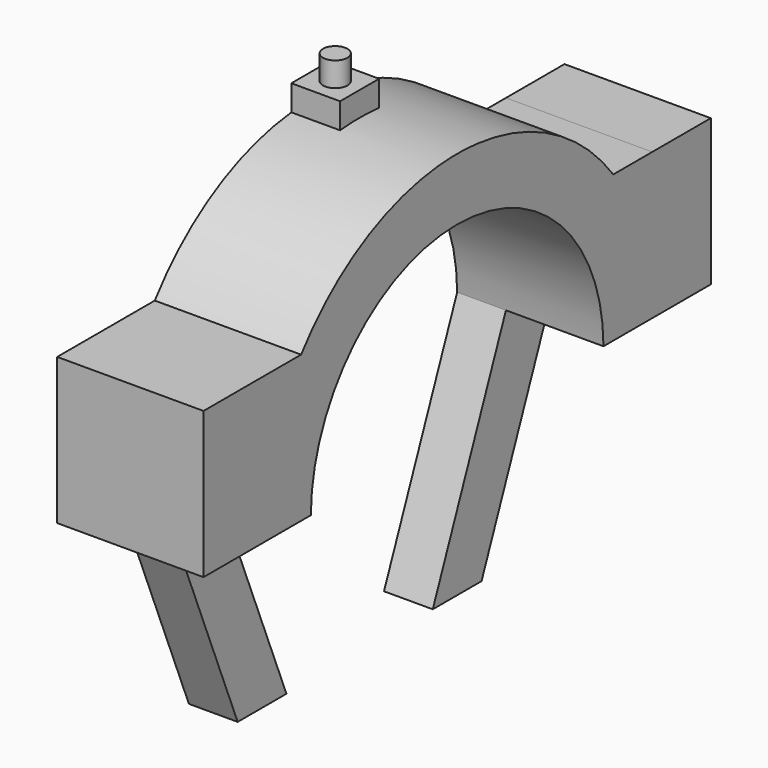
from build123d import *

# Parameters (mm, degrees)
F0_W     = 7.62
F0_H     = 15.24
F1_DEPTH = 5.08
F2_R     = 1.27
F3_DEPTH = 2.54
F4_DEPTH = 15.24


# Not quite as in the source:
# - ends of sketch curves that miss each other by under 0.0002 mm in the source are joined


with BuildPart() as f1:
    # F0 (on Right) → F1 (new body)
    with BuildSketch(Plane.YZ):
        Polygon((9.5176697043, 34.8342186189), (3.1676697043, 34.8342186189), (-6.3573302957, 11.2877884223), (-0.0073302957, 11.2877884223), align=None)
        with BuildLine():
            ThreePointArc((4.4376274036, 50.074186893), (8.2142139606, 42.8663955151), (9.5176697043, 34.8342186189))
            Line((9.5176697043, 34.8342186189), (9.5176697043, 50.0742186189))
            Line((9.5176697043, 50.0742186189), (4.4376274036, 50.074186893))
        make_face()
        with Locations((13.3276697043, 42.4542186189)):
            Rectangle(F0_W, F0_H)
        Polygon((-48.9023302957, 50.0742186189), (-48.9023302957, 34.8342186189), (-41.2823302957, 34.8342186189), (-41.28180154, 34.8342186189), (-41.28180154, 50.0742186189), align=None)
        with BuildLine():
            Line((-41.28180154, 50.0742186189), (-41.28180154, 34.8342186189))
            ThreePointArc((-41.28180154, 34.8342186189), (-39.9783395258, 42.8664143264), (-36.2017354445, 50.0742186189))
            Line((-36.2017354445, 50.0742186189), (-41.28180154, 50.0742186189))
        make_face()
        Polygon((-41.28180154, 34.8342186189), (-41.2823302957, 34.8342186189), (-31.7573302957, 11.2877884223), (-25.4073302957, 11.2877884223), (-34.9323302957, 34.8342186189), align=None)
        with BuildLine():
            ThreePointArc((-13.3423302957, 60.1066603814), (-15.8823316277, 60.2339542396), (-18.4223302957, 60.1066072389))
            Line((-18.4223302957, 60.1066072389), (-18.4223302957, 57.6942186189))
            Line((-18.4223302957, 57.6942186189), (-13.3423302957, 57.6942186189))
            Line((-13.3423302957, 57.6942186189), (-13.3423302957, 60.1066603814))
        make_face()
        with BuildLine():
            Line((-18.4223302957, 62.7742186189), (-18.4223302957, 60.1066072389))
            ThreePointArc((-18.4223302957, 60.1066072389), (-15.8823316277, 60.2339542396), (-13.3423302957, 60.1066603814))
            Line((-13.3423302957, 60.1066603814), (-13.3423302957, 62.7742186189))
            Line((-13.3423302957, 62.7742186189), (-18.4223302957, 62.7742186189))
        make_face()
        with BuildLine():
            ThreePointArc((-36.2017354445, 50.0742186189), (-39.9783395258, 42.8664143264), (-41.28180154, 34.8342186189))
            Line((-41.28180154, 34.8342186189), (-34.9323302957, 34.8342186189))
            ThreePointArc((-34.9323302957, 34.8342186189), (-15.8823302957, 53.7607736673), (3.1676697043, 34.8342186189))
            Line((3.1676697043, 34.8342186189), (9.5176697043, 34.8342186189))
            ThreePointArc((9.5176697043, 34.8342186189), (8.2142139606, 42.8663955151), (4.4376274036, 50.074186893))
            ThreePointArc((4.4376274036, 50.074186893), (-3.4000386794, 56.9553751368), (-13.3423302957, 60.1066603814))
            Line((-13.3423302957, 60.1066603814), (-13.3423302957, 57.6942186189))
            Line((-13.3423302957, 57.6942186189), (-18.4223302957, 57.6942186189))
            Line((-18.4223302957, 57.6942186189), (-18.4223302957, 60.1066072389))
            ThreePointArc((-18.4223302957, 60.1066072389), (-28.3643072986, 56.9552543041), (-36.2017354445, 50.0742186189))
        make_face()
    extrude(amount=F1_DEPTH)

    # F2 (on face) → F3 (join)
    with BuildSketch(Plane.XY.offset(62.7742186189)):
        with Locations((2.54, -15.8823302957)):
            Circle(F2_R)
    extrude(amount=F3_DEPTH)

    # F0 (on Right) → F4 (join)
    with BuildSketch(Plane.YZ):
        Polygon((-48.9023302957, 50.0742186189), (-48.9023302957, 34.8342186189), (-41.2823302957, 34.8342186189), (-41.28180154, 34.8342186189), (-41.28180154, 50.0742186189), align=None)
        with BuildLine():
            Line((-41.28180154, 50.0742186189), (-41.28180154, 34.8342186189))
            ThreePointArc((-41.28180154, 34.8342186189), (-39.9783395258, 42.8664143264), (-36.2017354445, 50.0742186189))
            Line((-36.2017354445, 50.0742186189), (-41.28180154, 50.0742186189))
        make_face()
        with BuildLine():
            ThreePointArc((-36.2017354445, 50.0742186189), (-39.9783395258, 42.8664143264), (-41.28180154, 34.8342186189))
            Line((-41.28180154, 34.8342186189), (-34.9323302957, 34.8342186189))
            ThreePointArc((-34.9323302957, 34.8342186189), (-15.8823302957, 53.7607736673), (3.1676697043, 34.8342186189))
            Line((3.1676697043, 34.8342186189), (9.5176697043, 34.8342186189))
            ThreePointArc((9.5176697043, 34.8342186189), (8.2142139606, 42.8663955151), (4.4376274036, 50.074186893))
            ThreePointArc((4.4376274036, 50.074186893), (-3.4000386794, 56.9553751368), (-13.3423302957, 60.1066603814))
            Line((-13.3423302957, 60.1066603814), (-13.3423302957, 57.6942186189))
            Line((-13.3423302957, 57.6942186189), (-18.4223302957, 57.6942186189))
            Line((-18.4223302957, 57.6942186189), (-18.4223302957, 60.1066072389))
            ThreePointArc((-18.4223302957, 60.1066072389), (-28.3643072986, 56.9552543041), (-36.2017354445, 50.0742186189))
        make_face()
        with BuildLine():
            ThreePointArc((4.4376274036, 50.074186893), (8.2142139606, 42.8663955151), (9.5176697043, 34.8342186189))
            Line((9.5176697043, 34.8342186189), (9.5176697043, 50.0742186189))
            Line((9.5176697043, 50.0742186189), (4.4376274036, 50.074186893))
        make_face()
        with Locations((13.3276697043, 42.4542186189)):
            Rectangle(F0_W, F0_H)
        with BuildLine():
            ThreePointArc((-13.3423302957, 60.1066603814), (-15.8823316277, 60.2339542396), (-18.4223302957, 60.1066072389))
            Line((-18.4223302957, 60.1066072389), (-18.4223302957, 57.6942186189))
            Line((-18.4223302957, 57.6942186189), (-13.3423302957, 57.6942186189))
            Line((-13.3423302957, 57.6942186189), (-13.3423302957, 60.1066603814))
        make_face()
    extrude(amount=F4_DEPTH)


solid = f1.part
